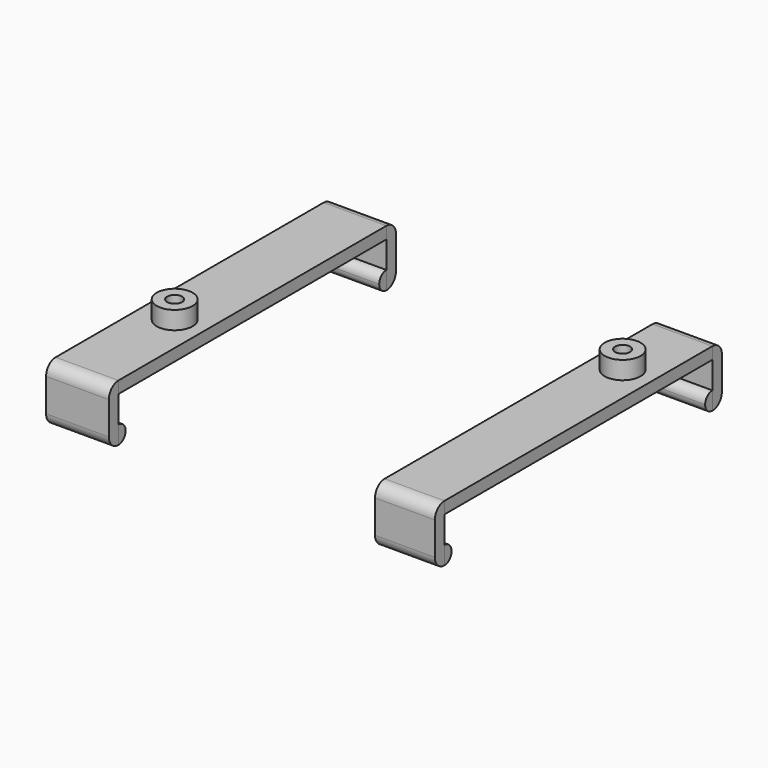
from build123d import *

# Parameters (mm, degrees)
F0_R     = 3
F0_R_2   = 1.25
F1_DEPTH = 5
F2_W     = 10.4999952316
F2_H     = 56
F3_DEPTH = 2
F2_W_2   = 10.0000047684
F4_W     = 10.4999952316
F4_H     = 2
F4_H_2   = 4.5
F4_H_3   = 3
F6_DEPTH = 2
F4_W_2   = 10.0000047684
F5_W     = 10.4999952316
F5_H     = 2
F5_H_2   = 4.5
F5_H_3   = 3
F7_DEPTH = 2
F5_W_2   = 10.0000047684
F5_H_4   = 6.5
F8_DEPTH = 1.5
F9_DEPTH = 1.5
F10_R    = 1.99999
F10_2_R  = 1.99999
F10_3_R  = 1.99999
F10_4_R  = 1.99999
F11_R    = 1.49999
F11_2_R  = 1.49999
F11_3_R  = 1.49999
F11_4_R  = 1.49999


# Not quite as in the source:
# - a fillet or chamfer is up to 0.001 mm smaller than in the source, because OpenCascade refuses the exact size


with BuildPart() as f1:
    # F0 (on Top) → F1 (new body)
    with BuildSketch(Plane.XY):
        with Locations((2.732144177, -27.8035767078)):
            Circle(F0_R)
        with Locations((2.732144177, -27.8035767078)):
            Circle(F0_R_2, mode=Mode.SUBTRACT)
    extrude(amount=F1_DEPTH)


with BuildPart() as f1b:
    # F0 (on Top) → F1, piece 2 (new body)
    with BuildSketch(Plane.XY):
        with Locations((57.232144177, -2.3035767078)):
            Circle(F0_R)
        with Locations((57.232144177, -2.3035767078)):
            Circle(F0_R_2, mode=Mode.SUBTRACT)
    extrude(amount=F1_DEPTH)


with BuildPart() as f3:
    # F2 (on Top) → F3 (new body)
    with BuildSketch(Plane.XY):
        with Locations((2.4821465611, -17.8035767078)):
            Rectangle(F2_W, F2_H)
    extrude(amount=F3_DEPTH)


with BuildPart() as f3b:
    # F2 (on Top) → F3, piece 2 (new body)
    with BuildSketch(Plane.XY):
        with Locations((57.2321465611, -17.8035767078)):
            Rectangle(F2_W_2, F2_H)
    extrude(amount=F3_DEPTH)


with BuildPart() as f6:
    # F4 (on face) → F6 (new body)
    with BuildSketch(Plane(origin=(0, 10.1964232922, 0), x_dir=(-1, 0, 0), z_dir=(0, 1, 0))):
        with Locations((-2.4821465611, 1)):
            Rectangle(F4_W, F4_H)
        with Locations((-2.4821465611, -2.25)):
            Rectangle(F4_W, F4_H_2)
        with Locations((-2.4821465611, -6)):
            Rectangle(F4_W, F4_H_3)
    extrude(amount=F6_DEPTH)

    # F10#3 (radius 2 in the source; OpenCascade refuses exactly that, so slightly less here)
    f10_3_edges = [f6.edges().sort_by_distance(p)[0] for p in [
        (2.482147, 12.196423, 2),
        (2.482147, 12.196423, -7.5),
    ]]
    fillet(f10_3_edges, radius=F10_3_R)


with BuildPart() as f6b:
    # F4 (on face) → F6, piece 2 (new body)
    with BuildSketch(Plane(origin=(0, 10.1964232922, 0), x_dir=(-1, 0, 0), z_dir=(0, 1, 0))):
        with Locations((-57.2321465611, 1)):
            Rectangle(F4_W_2, F4_H)
        with Locations((-57.2321465611, -2.25)):
            Rectangle(F4_W_2, F4_H_2)
        with Locations((-57.2321465611, -6)):
            Rectangle(F4_W_2, F4_H_3)
    extrude(amount=F6_DEPTH)

    # F10 (radius 2 in the source; OpenCascade refuses exactly that, so slightly less here)
    f10_edges = [f6b.edges().sort_by_distance(p)[0] for p in [
        (57.232147, 12.196423, 2),
        (57.232147, 12.196423, -7.5),
    ]]
    fillet(f10_edges, radius=F10_R)


with BuildPart() as f7:
    # F5 (on face) → F7 (new body)
    with BuildSketch(Plane.XZ.offset(45.8035767078)):
        with Locations((2.4821465611, 1)):
            Rectangle(F5_W, F5_H)
        with Locations((2.4821465611, -2.25)):
            Rectangle(F5_W, F5_H_2)
        with Locations((2.4821465611, -6)):
            Rectangle(F5_W, F5_H_3)
    extrude(amount=F7_DEPTH)

    # F10#4 (radius 2 in the source; OpenCascade refuses exactly that, so slightly less here)
    f10_4_edges = [f7.edges().sort_by_distance(p)[0] for p in [
        (2.482147, -47.803577, 2),
        (2.482147, -47.803577, -7.5),
    ]]
    fillet(f10_4_edges, radius=F10_4_R)


with BuildPart() as f7b:
    # F5 (on face) → F7, piece 2 (new body)
    with BuildSketch(Plane.XZ.offset(45.8035767078)):
        with Locations((57.2321465611, -1.25)):
            Rectangle(F5_W_2, F5_H_4)
        with Locations((57.2321465611, -6)):
            Rectangle(F5_W_2, F5_H_3)
    extrude(amount=F7_DEPTH)

    # F10#2 (radius 2 in the source; OpenCascade refuses exactly that, so slightly less here)
    f10_2_edges = [f7b.edges().sort_by_distance(p)[0] for p in [
        (57.232147, -47.803577, 2),
        (57.232147, -47.803577, -7.5),
    ]]
    fillet(f10_2_edges, radius=F10_2_R)


with BuildPart() as f8:
    # F4 (on face) → F8 (new body)
    with BuildSketch(Plane(origin=(0, 10.1964232922, 0), x_dir=(-1, 0, 0), z_dir=(0, 1, 0))):
        with Locations((-2.4821465611, -6)):
            Rectangle(F4_W, F4_H_3)
    extrude(amount=-F8_DEPTH)

    # F11#4 (radius 1.5 in the source; OpenCascade refuses exactly that, so slightly less here)
    f11_4_edges = [f8.edges().sort_by_distance(p)[0] for p in [
        (2.482147, 8.696423, -4.5),
        (2.482147, 8.696423, -7.5),
    ]]
    fillet(f11_4_edges, radius=F11_4_R)


with BuildPart() as f8b:
    # F4 (on face) → F8, piece 2 (new body)
    with BuildSketch(Plane(origin=(0, 10.1964232922, 0), x_dir=(-1, 0, 0), z_dir=(0, 1, 0))):
        with Locations((-57.2321465611, -6)):
            Rectangle(F4_W_2, F4_H_3)
    extrude(amount=-F8_DEPTH)

    # F11#3 (radius 1.5 in the source; OpenCascade refuses exactly that, so slightly less here)
    f11_3_edges = [f8b.edges().sort_by_distance(p)[0] for p in [
        (57.232147, 8.696423, -4.5),
        (57.232147, 8.696423, -7.5),
    ]]
    fillet(f11_3_edges, radius=F11_3_R)


with BuildPart() as f9:
    # F5 (on face) → F9 (new body)
    with BuildSketch(Plane.XZ.offset(45.8035767078)):
        with Locations((57.2321465611, -6)):
            Rectangle(F5_W_2, F5_H_3)
    extrude(amount=-F9_DEPTH)

    # F11#2 (radius 1.5 in the source; OpenCascade refuses exactly that, so slightly less here)
    f11_2_edges = [f9.edges().sort_by_distance(p)[0] for p in [
        (57.232147, -44.303577, -4.5),
        (57.232147, -44.303577, -7.5),
    ]]
    fillet(f11_2_edges, radius=F11_2_R)


with BuildPart() as f9b:
    # F5 (on face) → F9, piece 2 (new body)
    with BuildSketch(Plane.XZ.offset(45.8035767078)):
        with Locations((2.4821465611, -6)):
            Rectangle(F5_W, F5_H_3)
    extrude(amount=-F9_DEPTH)

    # F11 (radius 1.5 in the source; OpenCascade refuses exactly that, so slightly less here)
    f11_edges = [f9b.edges().sort_by_distance(p)[0] for p in [
        (2.482147, -44.303577, -7.5),
        (2.482147, -44.303577, -4.5),
    ]]
    fillet(f11_edges, radius=F11_R)


solid = Compound([f1.part, f1b.part, f3.part, f3b.part, f6.part, f6b.part, f7.part, f7b.part, f8.part, f8b.part, f9.part, f9b.part])
